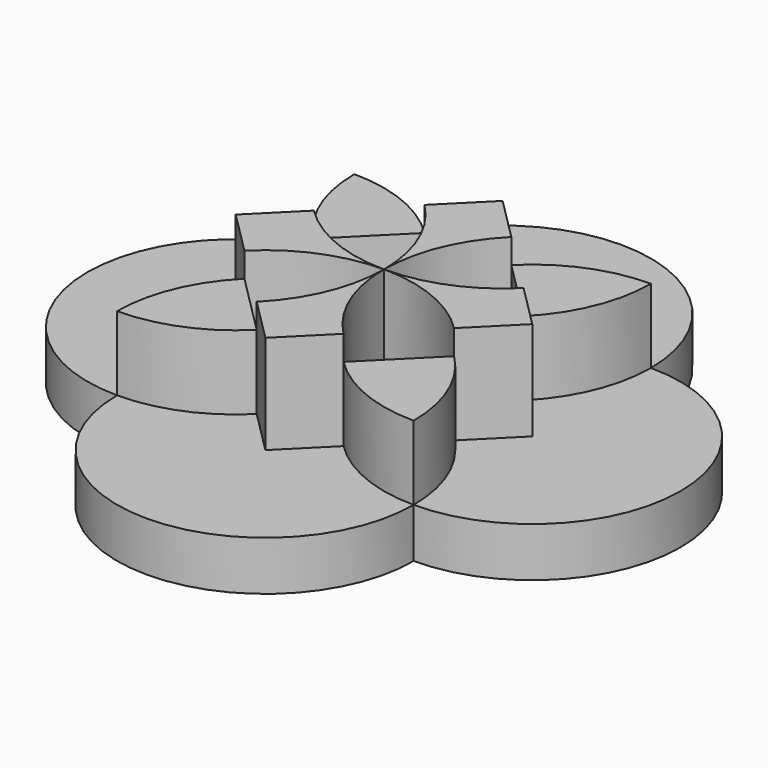
from build123d import *

# Parameters (mm, degrees)
F1_DEPTH = 25
F2_DEPTH = 10
F3_DEPTH = 30


with BuildPart() as f1:
    # F0 (on Top) → F1 (new body)
    with BuildSketch(Plane.XY):
        with BuildLine():
            ThreePointArc((21.2132034356, 8.7867965644), (27.7163859753, 18.519497029), (30, 30))
            ThreePointArc((30, 30), (18.519497029, 27.7163859753), (8.7867965644, 21.2132034356))
            Line((8.7867965644, 21.2132034356), (21.2132034356, 8.7867965644))
        make_face()
    extrude(amount=F1_DEPTH)


with BuildPart() as f1b:
    # F0 (on Top) → F1, piece 2 (new body)
    with BuildSketch(Plane.XY):
        with BuildLine():
            ThreePointArc((8.7867965644, -21.2132034356), (18.519497029, -27.7163859753), (30, -30))
            ThreePointArc((30, -30), (27.7163859753, -18.519497029), (21.2132034356, -8.7867965644))
            Line((21.2132034356, -8.7867965644), (8.7867965644, -21.2132034356))
        make_face()
    extrude(amount=F1_DEPTH)


with BuildPart() as f1c:
    # F0 (on Top) → F1, piece 3 (new body)
    with BuildSketch(Plane.XY):
        with BuildLine():
            ThreePointArc((-8.7867965644, 21.2132034356), (-18.519497029, 27.7163859753), (-30, 30))
            ThreePointArc((-30, 30), (-27.7163859753, 18.519497029), (-21.2132034356, 8.7867965644))
            Line((-21.2132034356, 8.7867965644), (-8.7867965644, 21.2132034356))
        make_face()
    extrude(amount=F1_DEPTH)


with BuildPart() as f1d:
    # F0 (on Top) → F1, piece 4 (new body)
    with BuildSketch(Plane.XY):
        with BuildLine():
            ThreePointArc((-21.2132034356, -8.7867965644), (-27.7163859753, -18.519497029), (-30, -30))
            ThreePointArc((-30, -30), (-18.519497029, -27.7163859753), (-8.7867965644, -21.2132034356))
            Line((-8.7867965644, -21.2132034356), (-21.2132034356, -8.7867965644))
        make_face()
    extrude(amount=F1_DEPTH)


with BuildPart() as f2:
    # F0 (on Top) → F2 (new body)
    with BuildSketch(Plane.XY):
        with BuildLine():
            ThreePointArc((30, -30), (51.2132034356, -21.2132034356), (60, 0))
            ThreePointArc((60, 0), (51.2132034356, 21.2132034356), (30, 30))
            ThreePointArc((30, 30), (27.7163859753, 18.519497029), (21.2132034356, 8.7867965644))
            Line((21.2132034356, 8.7867965644), (30, 0))
            Line((30, 0), (21.2132034356, -8.7867965644))
            ThreePointArc((21.2132034356, -8.7867965644), (27.7163859753, -18.519497029), (30, -30))
        make_face()
    extrude(amount=F2_DEPTH)


with BuildPart() as f2b:
    # F0 (on Top) → F2, piece 2 (new body)
    with BuildSketch(Plane.XY):
        with BuildLine():
            ThreePointArc((8.7867965644, 21.2132034356), (18.519497029, 27.7163859753), (30, 30))
            ThreePointArc((30, 30), (0, 60), (-30, 30))
            ThreePointArc((-30, 30), (-18.519497029, 27.7163859753), (-8.7867965644, 21.2132034356))
            Line((-8.7867965644, 21.2132034356), (0, 30))
            Line((0, 30), (8.7867965644, 21.2132034356))
        make_face()
    extrude(amount=F2_DEPTH)


with BuildPart() as f2c:
    # F0 (on Top) → F2, piece 3 (new body)
    with BuildSketch(Plane.XY):
        with BuildLine():
            ThreePointArc((-30, -30), (0, -60), (30, -30))
            ThreePointArc((30, -30), (18.519497029, -27.7163859753), (8.7867965644, -21.2132034356))
            Line((8.7867965644, -21.2132034356), (0, -30))
            Line((0, -30), (-8.7867965644, -21.2132034356))
            ThreePointArc((-8.7867965644, -21.2132034356), (-18.519497029, -27.7163859753), (-30, -30))
        make_face()
    extrude(amount=F2_DEPTH)


with BuildPart() as f2d:
    # F0 (on Top) → F2, piece 4 (new body)
    with BuildSketch(Plane.XY):
        with BuildLine():
            ThreePointArc((-21.2132034356, 8.7867965644), (-27.7163859753, 18.519497029), (-30, 30))
            ThreePointArc((-30, 30), (-60, 0), (-30, -30))
            ThreePointArc((-30, -30), (-27.7163859753, -18.519497029), (-21.2132034356, -8.7867965644))
            Line((-21.2132034356, -8.7867965644), (-30, 0))
            Line((-30, 0), (-21.2132034356, 8.7867965644))
        make_face()
    extrude(amount=F2_DEPTH)


with BuildPart() as f3:
    # F0 (on Top) → F3 (new body)
    with BuildSketch(Plane.XY):
        with BuildLine():
            ThreePointArc((0, 0), (2.2836140247, 11.480502971), (8.7867965644, 21.2132034356))
            Line((8.7867965644, 21.2132034356), (0, 30))
            Line((0, 30), (-8.7867965644, 21.2132034356))
            ThreePointArc((-8.7867965644, 21.2132034356), (-2.2836140247, 11.480502971), (0, 0))
        make_face()
    extrude(amount=F3_DEPTH)


with BuildPart() as f3b:
    # F0 (on Top) → F3, piece 2 (new body)
    with BuildSketch(Plane.XY):
        with BuildLine():
            Line((0, -30), (8.7867965644, -21.2132034356))
            ThreePointArc((8.7867965644, -21.2132034356), (2.2836140247, -11.480502971), (0, 0))
            ThreePointArc((0, 0), (-2.2836140247, -11.480502971), (-8.7867965644, -21.2132034356))
            Line((-8.7867965644, -21.2132034356), (0, -30))
        make_face()
    extrude(amount=F3_DEPTH)


with BuildPart() as f3c:
    # F0 (on Top) → F3, piece 3 (new body)
    with BuildSketch(Plane.XY):
        with BuildLine():
            ThreePointArc((-21.2132034356, -8.7867965644), (-11.480502971, -2.2836140247), (0, 0))
            ThreePointArc((0, 0), (-11.480502971, 2.2836140247), (-21.2132034356, 8.7867965644))
            Line((-21.2132034356, 8.7867965644), (-30, 0))
            Line((-30, 0), (-21.2132034356, -8.7867965644))
        make_face()
    extrude(amount=F3_DEPTH)


with BuildPart() as f3d:
    # F0 (on Top) → F3, piece 4 (new body)
    with BuildSketch(Plane.XY):
        with BuildLine():
            Line((30, 0), (21.2132034356, 8.7867965644))
            ThreePointArc((21.2132034356, 8.7867965644), (11.480502971, 2.2836140247), (0, 0))
            ThreePointArc((0, 0), (11.480502971, -2.2836140247), (21.2132034356, -8.7867965644))
            Line((21.2132034356, -8.7867965644), (30, 0))
        make_face()
    extrude(amount=F3_DEPTH)


solid = Compound([f1.part, f1b.part, f1c.part, f1d.part, f2.part, f2b.part, f2c.part, f2d.part, f3.part, f3b.part, f3c.part, f3d.part])
